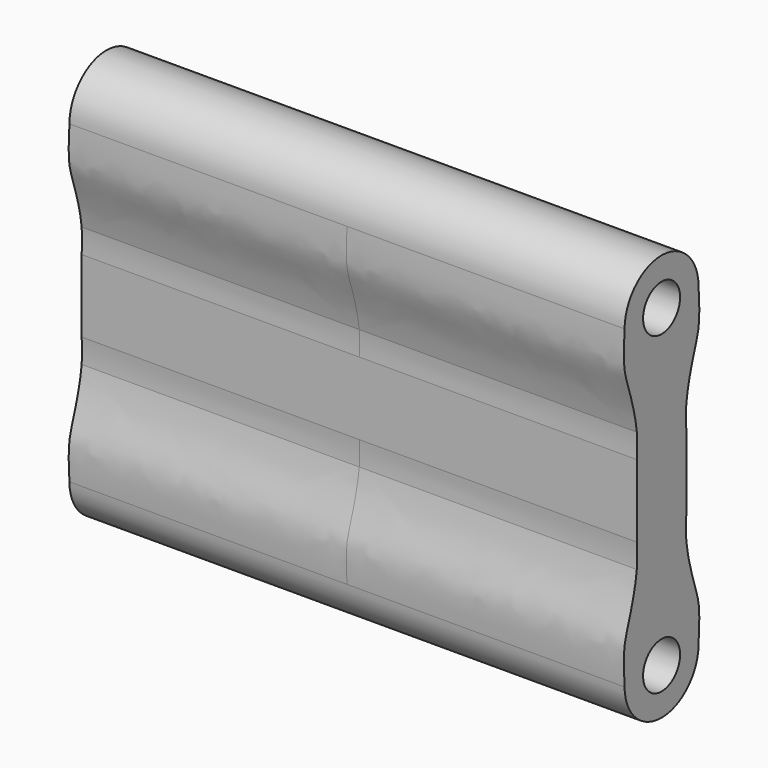
from build123d import *

# Parameters (mm, degrees)
F0_R     = 6.35
F1_DEPTH = 76.2


with BuildPart() as f1:
    # F0 (on Right) → F1 (new body, symmetric)
    with BuildSketch(Plane.YZ):
        with BuildLine():
            ThreePointArc((-12.6997439282, 43.2606483645), (-0.0403243855, 30.4800640181), (12.7, 43.18))
            ThreePointArc((12.7, 43.18), (12.6999359819, 43.2203243855), (12.6997439282, 43.2606483645))
            ThreePointArc((12.6997439282, 43.2606483645), (0, 55.88), (-12.6997439282, 43.2606483645))
        make_face()
        with Locations((0, 43.18)):
            Circle(F0_R, mode=Mode.SUBTRACT)
        with BuildLine():
            ThreePointArc((12.6997439282, 43.2606483645), (12.6999359819, 43.2203243855), (12.7, 43.18))
            ThreePointArc((12.7, 43.18), (-0.0403243855, 30.4800640181), (-12.6997439282, 43.2606483645))
            add(Edge.make_bspline(
                [(-12.6997439282, 43.2606483645), (-12.8988694733, 39.9507329366), (-13.2741153741, 33.8014875907), (-11.0697013918, 27.9600935569), (-8.8773627451, 20.2984769123), (-8.4960911469, 16.6054463091)],
                knots=[0, 0, 0, 0, 0.2069133804, 0.3779212986, 0.608638832, 0.608638832, 0.608638832, 0.608638832], degree=3))
            add(Edge.make_bspline(
                [(-8.4960911469, 16.6054463091), (-8.2450556241, 14.1738939135), (-8.3745678607, 12.0489048905), (-8.4960911469, 9.9725638339)],
                knots=[0.608638832, 0.608638832, 0.608638832, 0.608638832, 0.7605470698, 0.7605470698, 0.7605470698, 0.7605470698], degree=3))
            Line((-8.4960911469, 9.9725638339), (-8.4960911469, -9.9725638339))
            add(Edge.make_bspline(
                [(-8.4960911469, -16.6054463091), (-8.2450556241, -14.1738939135), (-8.3745678607, -12.0489048905), (-8.4960911469, -9.9725638339)],
                knots=[0.608638832, 0.608638832, 0.608638832, 0.608638832, 0.7605470698, 0.7605470698, 0.7605470698, 0.7605470698], degree=3))
            add(Edge.make_bspline(
                [(-12.6997439282, -43.2606483645), (-12.8988694733, -39.9507329366), (-13.2741153741, -33.8014875907), (-11.0697013918, -27.9600935569), (-8.8773627451, -20.2984769123), (-8.4960911469, -16.6054463091)],
                knots=[0, 0, 0, 0, 0.2069133804, 0.3779212986, 0.608638832, 0.608638832, 0.608638832, 0.608638832], degree=3))
            ThreePointArc((-12.6997439282, -43.2606483645), (-0.0403243855, -30.4800640181), (12.7, -43.18))
            ThreePointArc((12.7, -43.18), (12.6999359819, -43.2203243855), (12.6997439282, -43.2606483645))
            add(Edge.make_bspline(
                [(12.6997439282, -43.2606483645), (12.8988694733, -39.9507329366), (13.2741153741, -33.8014875907), (11.0697013918, -27.9600935569), (7.7953126844, -16.5170115042), (8.4890847839, -10.7802367673), (8.5940876598, -8.0775288451)],
                knots=[0, 0, 0, 0, 0.2069133804, 0.3779212986, 0.608638832, 0.8069143356, 0.8069143356, 0.8069143356, 0.8069143356], degree=3))
            Line((8.5940876598, -8.0775288451), (8.5243625131, 9.4845660853))
            add(Edge.make_bspline(
                [(8.4960911469, 16.6054463091), (8.2253576614, 13.9830976955), (8.3972357404, 11.7173100932), (8.5243625131, 9.4845660853)],
                knots=[0.608638832, 0.608638832, 0.608638832, 0.608638832, 0.7724668282, 0.7724668282, 0.7724668282, 0.7724668282], degree=3))
            add(Edge.make_bspline(
                [(12.6997439282, 43.2606483645), (12.8988694733, 39.9507329366), (13.2741153741, 33.8014875907), (11.0697013918, 27.9600935569), (8.8773627451, 20.2984769123), (8.4960911469, 16.6054463091)],
                knots=[0, 0, 0, 0, 0.2069133804, 0.3779212986, 0.608638832, 0.608638832, 0.608638832, 0.608638832], degree=3))
        make_face()
        with BuildLine():
            ThreePointArc((-12.6997439282, -43.2606483645), (0, -55.88), (12.6997439282, -43.2606483645))
            ThreePointArc((12.6997439282, -43.2606483645), (12.6999359819, -43.2203243855), (12.7, -43.18))
            ThreePointArc((12.7, -43.18), (-0.0403243855, -30.4800640181), (-12.6997439282, -43.2606483645))
        make_face()
        with Locations((0, -43.18)):
            Circle(F0_R, mode=Mode.SUBTRACT)
    extrude(amount=F1_DEPTH, both=True)


solid = f1.part
